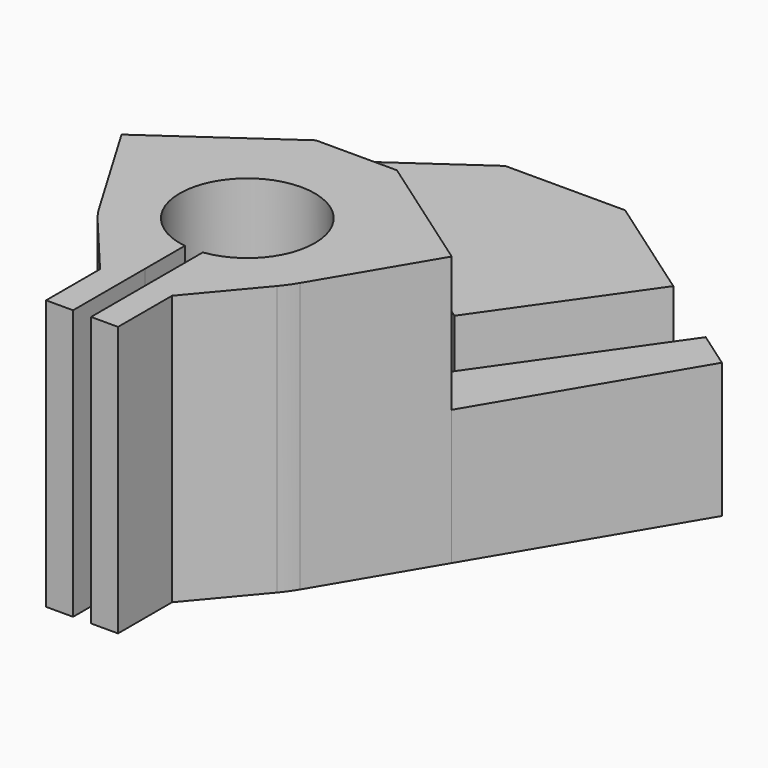
from build123d import *

# Parameters (mm, degrees)
F1_W     = 1.45
F1_H     = 6.3409252325
F2_DEPTH = 5
F3_DEPTH = 10
F5_DEPTH = 25
F6_DEPTH = 10
F4_R     = 0.725
F7_DEPTH = 32.664992266
F4_R_2   = 1.025
F8_DEPTH = 20.2234430885


# Not quite as in the source:
# - a feature names something its author has since deleted; it is built from what else it names


with BuildPart() as f2:
    # F1 (on Top) → F2 (new body)
    with BuildSketch(Plane.XY):
        with BuildLine():
            ThreePointArc((-21.8973851311, -18.9294214119), (-28.3829246015, -10.9960880786), (-20.899609828, -3.9960880786))
            ThreePointArc((-20.899609828, -3.9960880786), (-13.4162950544, -10.9960880786), (-19.9018345249, -18.9294214119))
            Line((-19.9018345249, -18.9294214119), (-19.9003497467, -24.4576265402))
            ThreePointArc((-19.9003497467, -24.4576265402), (-18.3828834375, -24.250149717), (-16.9003497467, -23.8656442066))
            ThreePointArc((-16.9003497467, -23.8656442066), (-13.6367119074, -22.2780319569), (-10.9391436703, -19.8500759839))
            ThreePointArc((-10.9391436703, -19.8500759839), (-10.2927451499, -19.0123651957), (-9.7166149372, -18.12486061))
            ThreePointArc((-9.7166149372, -18.12486061), (-9.4290474991, -5.3783924455), (-20.174609828, 1.4836798315))
            Line((-20.174609828, 1.4836798315), (-20.174609828, 0))
            Line((-20.174609828, 0), (-20.899609828, 0))
            Line((-20.899609828, 0), (-21.624609828, 0))
            Line((-21.624609828, 0), (-21.624609828, 1.4836798315))
            ThreePointArc((-21.624609828, 1.4836798315), (-32.3701721569, -5.3783924455), (-32.0826047188, -18.12486061))
            ThreePointArc((-32.0826047188, -18.12486061), (-31.5064745061, -19.0123651957), (-30.8600759857, -19.8500759839))
            ThreePointArc((-30.8600759857, -19.8500759839), (-28.1625077486, -22.2780319569), (-24.8988699093, -23.8656442066))
            ThreePointArc((-24.8988699093, -23.8656442066), (-23.4163362185, -24.250149717), (-21.8988699093, -24.4576265402))
            Line((-21.8988699093, -24.4576265402), (-21.8973851311, -18.9294214119))
        make_face()
        with BuildLine():
            Line((-21.8988699093, -34.4576265402), (-21.8988699093, -24.4576265402))
            ThreePointArc((-21.8988699093, -24.4576265402), (-23.4163362185, -24.250149717), (-24.8988699093, -23.8656442066))
            Line((-24.8988699093, -23.8656442066), (-24.8988699093, -26.9576265402))
            Line((-24.8988699093, -26.9576265402), (-24.8988699093, -34.4576265402))
            Line((-24.8988699093, -34.4576265402), (-21.8988699093, -34.4576265402))
        make_face()
        with BuildLine():
            ThreePointArc((-16.9003497467, -23.8656442066), (-18.3828834375, -24.250149717), (-19.9003497467, -24.4576265402))
            Line((-19.9003497467, -24.4576265402), (-19.9003497467, -34.4576265402))
            Line((-19.9003497467, -34.4576265402), (-16.9003497467, -34.4576265402))
            Line((-16.9003497467, -34.4576265402), (-16.9003497467, -26.9576265402))
            Line((-16.9003497467, -26.9576265402), (-16.9003497467, -23.8656442066))
        make_face()
        with BuildLine():
            Line((-24.8988699093, -26.9576265402), (-24.8988699093, -23.8656442066))
            ThreePointArc((-24.8988699093, -23.8656442066), (-28.1625077486, -22.2780319569), (-30.8600759857, -19.8500759839))
            Line((-30.8600759857, -19.8500759839), (-24.8988699093, -26.9576265402))
        make_face()
        with BuildLine():
            ThreePointArc((-10.9391436703, -19.8500759839), (-13.6367119074, -22.2780319569), (-16.9003497467, -23.8656442066))
            Line((-16.9003497467, -23.8656442066), (-16.9003497467, -26.9576265402))
            Line((-16.9003497467, -26.9576265402), (-10.9391436703, -19.8500759839))
        make_face()
        with BuildLine():
            Line((-39.2498481908, -6.0334444768), (-32.0826047188, -18.12486061))
            ThreePointArc((-32.0826047188, -18.12486061), (-32.3701721569, -5.3783924455), (-21.624609828, 1.4836798315))
            Line((-21.624609828, 1.4836798315), (-21.624609828, 3.6590747675))
            Line((-21.624609828, 3.6590747675), (-25.4074961518, 3.6590747675))
            Line((-25.4074961518, 3.6590747675), (-33.5990165947, -2.076689596))
            Line((-33.5990165947, -2.076689596), (-39.2498481908, -6.0334444768))
        make_face()
        with BuildLine():
            ThreePointArc((-20.174609828, 1.4836798315), (-9.4290474991, -5.3783924455), (-9.7166149372, -18.12486061))
            Line((-9.7166149372, -18.12486061), (-2.5493714652, -6.0334444768))
            Line((-2.5493714652, -6.0334444768), (-8.2002030613, -2.076689596))
            Line((-8.2002030613, -2.076689596), (-16.3917235042, 3.6590747675))
            Line((-16.3917235042, 3.6590747675), (-20.174609828, 3.6590747675))
            Line((-20.174609828, 3.6590747675), (-20.174609828, 1.4836798315))
        make_face()
        with BuildLine():
            Line((-21.624609828, 3.6590747675), (-21.624609828, 1.4836798315))
            ThreePointArc((-21.624609828, 1.4836798315), (-21.2622509514, 1.4988529145), (-20.899609828, 1.5039119214))
            ThreePointArc((-20.899609828, 1.5039119214), (-20.5369687046, 1.4988529145), (-20.174609828, 1.4836798315))
            Line((-20.174609828, 1.4836798315), (-20.174609828, 3.6590747675))
            Line((-20.174609828, 3.6590747675), (-21.624609828, 3.6590747675))
        make_face()
        with BuildLine():
            ThreePointArc((-20.899609828, 1.5039119214), (-21.2622509514, 1.4988529145), (-21.624609828, 1.4836798315))
            Line((-21.624609828, 1.4836798315), (-21.624609828, 0))
            Line((-21.624609828, 0), (-20.899609828, 0))
            Line((-20.899609828, 0), (-20.174609828, 0))
            Line((-20.174609828, 0), (-20.174609828, 1.4836798315))
            ThreePointArc((-20.174609828, 1.4836798315), (-20.5369687046, 1.4988529145), (-20.899609828, 1.5039119214))
        make_face()
        Polygon((-52.0341877249, 15.5342293294), (-39.2498481908, -6.0334444768), (-33.5990165947, -2.076689596), (-47.9384275035, 18.4021115112), align=None)
        Polygon((-8.2002030613, -2.076689596), (-2.5493714652, -6.0334444768), (10.2349680689, 15.5342293294), (6.1392078475, 18.4021115112), align=None)
        Polygon((-25.4074961518, 3.6590747675), (-21.624609828, 3.6590747675), (-21.624609828, 10), (-21.924609828, 10), (-27.2409219547, 6.2774781734), align=None)
        with Locations((-20.899609828, 6.8295373837)):
            Rectangle(F1_W, F1_H)
        Polygon((-47.9384275035, 18.4021115112), (-33.5990165947, -2.076689596), (-25.4074961518, 3.6590747675), (-27.2409219547, 6.2774781734), (-28.3880748274, 7.915782262), (-39.7469070606, 24.1378758747), align=None)
        Polygon((-16.3917235042, 3.6590747675), (-8.2002030613, -2.076689596), (6.1392078475, 18.4021115112), (-2.0523125954, 24.1378758747), (-13.4111448286, 7.915782262), (-14.5582977013, 6.2774781734), align=None)
        Polygon((-20.174609828, 10), (-20.174609828, 3.6590747675), (-16.3917235042, 3.6590747675), (-14.5582977013, 6.2774781734), (-19.874609828, 10), align=None)
        Polygon((-21.924609828, 10), (-21.624609828, 10), (-20.174609828, 10), (-19.874609828, 10), (-19.874609828, 12.4415491775), (-21.924609828, 12.4415491775), align=None)
        Polygon((-27.2409219547, 6.2774781734), (-21.924609828, 10), (-21.924609828, 12.4415491775), (-27.5689227831, 8.4893586983), (-28.3880748274, 7.915782262), align=None)
        Polygon((-38.9277550163, 24.7114523111), (-39.7469070606, 24.1378758747), (-28.3880748274, 7.915782262), (-27.5689227831, 8.4893586983), (-27.5689227831, 32.664992266), align=None)
        Polygon((-13.4111448286, 7.915782262), (-2.0523125954, 24.1378758747), (-2.8714646397, 24.7114523111), (-14.2302968729, 32.664992266), (-14.2302968729, 8.4893586983), align=None)
        Polygon((-19.874609828, 10), (-14.5582977013, 6.2774781734), (-13.4111448286, 7.915782262), (-14.2302968729, 8.4893586983), (-19.874609828, 12.4415491775), align=None)
        Polygon((-27.5689227831, 8.4893586983), (-21.924609828, 12.4415491775), (-21.924609828, 32.664992266), (-27.5689227831, 32.664992266), align=None)
        Polygon((-21.924609828, 32.664992266), (-21.924609828, 12.4415491775), (-19.874609828, 12.4415491775), (-19.874609828, 32.664992266), (-20.899609828, 32.664992266), align=None)
        Polygon((-19.874609828, 32.664992266), (-19.874609828, 12.4415491775), (-14.2302968729, 8.4893586983), (-14.2302968729, 32.664992266), align=None)
    extrude(amount=-F2_DEPTH)

    # F1 (on Top) → F5 (join)
    with BuildSketch(Plane.XY):
        with BuildLine():
            ThreePointArc((-21.8973851311, -18.9294214119), (-28.3829246015, -10.9960880786), (-20.899609828, -3.9960880786))
            ThreePointArc((-20.899609828, -3.9960880786), (-13.4162950544, -10.9960880786), (-19.9018345249, -18.9294214119))
            Line((-19.9018345249, -18.9294214119), (-19.9003497467, -24.4576265402))
            ThreePointArc((-19.9003497467, -24.4576265402), (-18.3828834375, -24.250149717), (-16.9003497467, -23.8656442066))
            ThreePointArc((-16.9003497467, -23.8656442066), (-13.6367119074, -22.2780319569), (-10.9391436703, -19.8500759839))
            ThreePointArc((-10.9391436703, -19.8500759839), (-10.2927451499, -19.0123651957), (-9.7166149372, -18.12486061))
            ThreePointArc((-9.7166149372, -18.12486061), (-9.4290474991, -5.3783924455), (-20.174609828, 1.4836798315))
            Line((-20.174609828, 1.4836798315), (-20.174609828, 0))
            Line((-20.174609828, 0), (-20.899609828, 0))
            Line((-20.899609828, 0), (-21.624609828, 0))
            Line((-21.624609828, 0), (-21.624609828, 1.4836798315))
            ThreePointArc((-21.624609828, 1.4836798315), (-32.3701721569, -5.3783924455), (-32.0826047188, -18.12486061))
            ThreePointArc((-32.0826047188, -18.12486061), (-31.5064745061, -19.0123651957), (-30.8600759857, -19.8500759839))
            ThreePointArc((-30.8600759857, -19.8500759839), (-28.1625077486, -22.2780319569), (-24.8988699093, -23.8656442066))
            ThreePointArc((-24.8988699093, -23.8656442066), (-23.4163362185, -24.250149717), (-21.8988699093, -24.4576265402))
            Line((-21.8988699093, -24.4576265402), (-21.8973851311, -18.9294214119))
        make_face()
        with BuildLine():
            Line((-21.8988699093, -34.4576265402), (-21.8988699093, -24.4576265402))
            ThreePointArc((-21.8988699093, -24.4576265402), (-23.4163362185, -24.250149717), (-24.8988699093, -23.8656442066))
            Line((-24.8988699093, -23.8656442066), (-24.8988699093, -26.9576265402))
            Line((-24.8988699093, -26.9576265402), (-24.8988699093, -34.4576265402))
            Line((-24.8988699093, -34.4576265402), (-21.8988699093, -34.4576265402))
        make_face()
        with BuildLine():
            ThreePointArc((-16.9003497467, -23.8656442066), (-18.3828834375, -24.250149717), (-19.9003497467, -24.4576265402))
            Line((-19.9003497467, -24.4576265402), (-19.9003497467, -34.4576265402))
            Line((-19.9003497467, -34.4576265402), (-16.9003497467, -34.4576265402))
            Line((-16.9003497467, -34.4576265402), (-16.9003497467, -26.9576265402))
            Line((-16.9003497467, -26.9576265402), (-16.9003497467, -23.8656442066))
        make_face()
        with BuildLine():
            Line((-24.8988699093, -26.9576265402), (-24.8988699093, -23.8656442066))
            ThreePointArc((-24.8988699093, -23.8656442066), (-28.1625077486, -22.2780319569), (-30.8600759857, -19.8500759839))
            Line((-30.8600759857, -19.8500759839), (-24.8988699093, -26.9576265402))
        make_face()
        with BuildLine():
            ThreePointArc((-10.9391436703, -19.8500759839), (-13.6367119074, -22.2780319569), (-16.9003497467, -23.8656442066))
            Line((-16.9003497467, -23.8656442066), (-16.9003497467, -26.9576265402))
            Line((-16.9003497467, -26.9576265402), (-10.9391436703, -19.8500759839))
        make_face()
        with BuildLine():
            Line((-39.2498481908, -6.0334444768), (-32.0826047188, -18.12486061))
            ThreePointArc((-32.0826047188, -18.12486061), (-32.3701721569, -5.3783924455), (-21.624609828, 1.4836798315))
            Line((-21.624609828, 1.4836798315), (-21.624609828, 3.6590747675))
            Line((-21.624609828, 3.6590747675), (-25.4074961518, 3.6590747675))
            Line((-25.4074961518, 3.6590747675), (-33.5990165947, -2.076689596))
            Line((-33.5990165947, -2.076689596), (-39.2498481908, -6.0334444768))
        make_face()
        with BuildLine():
            ThreePointArc((-20.174609828, 1.4836798315), (-9.4290474991, -5.3783924455), (-9.7166149372, -18.12486061))
            Line((-9.7166149372, -18.12486061), (-2.5493714652, -6.0334444768))
            Line((-2.5493714652, -6.0334444768), (-8.2002030613, -2.076689596))
            Line((-8.2002030613, -2.076689596), (-16.3917235042, 3.6590747675))
            Line((-16.3917235042, 3.6590747675), (-20.174609828, 3.6590747675))
            Line((-20.174609828, 3.6590747675), (-20.174609828, 1.4836798315))
        make_face()
        with BuildLine():
            Line((-21.624609828, 3.6590747675), (-21.624609828, 1.4836798315))
            ThreePointArc((-21.624609828, 1.4836798315), (-21.2622509514, 1.4988529145), (-20.899609828, 1.5039119214))
            ThreePointArc((-20.899609828, 1.5039119214), (-20.5369687046, 1.4988529145), (-20.174609828, 1.4836798315))
            Line((-20.174609828, 1.4836798315), (-20.174609828, 3.6590747675))
            Line((-20.174609828, 3.6590747675), (-21.624609828, 3.6590747675))
        make_face()
        with BuildLine():
            ThreePointArc((-20.899609828, 1.5039119214), (-21.2622509514, 1.4988529145), (-21.624609828, 1.4836798315))
            Line((-21.624609828, 1.4836798315), (-21.624609828, 0))
            Line((-21.624609828, 0), (-20.899609828, 0))
            Line((-20.899609828, 0), (-20.174609828, 0))
            Line((-20.174609828, 0), (-20.174609828, 1.4836798315))
            ThreePointArc((-20.174609828, 1.4836798315), (-20.5369687046, 1.4988529145), (-20.899609828, 1.5039119214))
        make_face()
    extrude(amount=F5_DEPTH)

    # F1 (on Top) → F6 (join)
    with BuildSketch(Plane.XY):
        with BuildLine():
            ThreePointArc((-21.8973851311, -18.9294214119), (-28.3829246015, -10.9960880786), (-20.899609828, -3.9960880786))
            ThreePointArc((-20.899609828, -3.9960880786), (-13.4162950544, -10.9960880786), (-19.9018345249, -18.9294214119))
            Line((-19.9018345249, -18.9294214119), (-19.9003497467, -24.4576265402))
            ThreePointArc((-19.9003497467, -24.4576265402), (-18.3828834375, -24.250149717), (-16.9003497467, -23.8656442066))
            ThreePointArc((-16.9003497467, -23.8656442066), (-13.6367119074, -22.2780319569), (-10.9391436703, -19.8500759839))
            ThreePointArc((-10.9391436703, -19.8500759839), (-10.2927451499, -19.0123651957), (-9.7166149372, -18.12486061))
            ThreePointArc((-9.7166149372, -18.12486061), (-9.4290474991, -5.3783924455), (-20.174609828, 1.4836798315))
            Line((-20.174609828, 1.4836798315), (-20.174609828, 0))
            Line((-20.174609828, 0), (-20.899609828, 0))
            Line((-20.899609828, 0), (-21.624609828, 0))
            Line((-21.624609828, 0), (-21.624609828, 1.4836798315))
            ThreePointArc((-21.624609828, 1.4836798315), (-32.3701721569, -5.3783924455), (-32.0826047188, -18.12486061))
            ThreePointArc((-32.0826047188, -18.12486061), (-31.5064745061, -19.0123651957), (-30.8600759857, -19.8500759839))
            ThreePointArc((-30.8600759857, -19.8500759839), (-28.1625077486, -22.2780319569), (-24.8988699093, -23.8656442066))
            ThreePointArc((-24.8988699093, -23.8656442066), (-23.4163362185, -24.250149717), (-21.8988699093, -24.4576265402))
            Line((-21.8988699093, -24.4576265402), (-21.8973851311, -18.9294214119))
        make_face()
        with BuildLine():
            Line((-24.8988699093, -26.9576265402), (-24.8988699093, -23.8656442066))
            ThreePointArc((-24.8988699093, -23.8656442066), (-28.1625077486, -22.2780319569), (-30.8600759857, -19.8500759839))
            Line((-30.8600759857, -19.8500759839), (-24.8988699093, -26.9576265402))
        make_face()
        with BuildLine():
            Line((-21.8988699093, -34.4576265402), (-21.8988699093, -24.4576265402))
            ThreePointArc((-21.8988699093, -24.4576265402), (-23.4163362185, -24.250149717), (-24.8988699093, -23.8656442066))
            Line((-24.8988699093, -23.8656442066), (-24.8988699093, -26.9576265402))
            Line((-24.8988699093, -26.9576265402), (-24.8988699093, -34.4576265402))
            Line((-24.8988699093, -34.4576265402), (-21.8988699093, -34.4576265402))
        make_face()
        with BuildLine():
            ThreePointArc((-16.9003497467, -23.8656442066), (-18.3828834375, -24.250149717), (-19.9003497467, -24.4576265402))
            Line((-19.9003497467, -24.4576265402), (-19.9003497467, -34.4576265402))
            Line((-19.9003497467, -34.4576265402), (-16.9003497467, -34.4576265402))
            Line((-16.9003497467, -34.4576265402), (-16.9003497467, -26.9576265402))
            Line((-16.9003497467, -26.9576265402), (-16.9003497467, -23.8656442066))
        make_face()
        with BuildLine():
            ThreePointArc((-10.9391436703, -19.8500759839), (-13.6367119074, -22.2780319569), (-16.9003497467, -23.8656442066))
            Line((-16.9003497467, -23.8656442066), (-16.9003497467, -26.9576265402))
            Line((-16.9003497467, -26.9576265402), (-10.9391436703, -19.8500759839))
        make_face()
        Polygon((-52.0341877249, 15.5342293294), (-39.2498481908, -6.0334444768), (-33.5990165947, -2.076689596), (-47.9384275035, 18.4021115112), align=None)
        Polygon((-8.2002030613, -2.076689596), (-2.5493714652, -6.0334444768), (10.2349680689, 15.5342293294), (6.1392078475, 18.4021115112), align=None)
        with BuildLine():
            Line((-39.2498481908, -6.0334444768), (-32.0826047188, -18.12486061))
            ThreePointArc((-32.0826047188, -18.12486061), (-32.3701721569, -5.3783924455), (-21.624609828, 1.4836798315))
            Line((-21.624609828, 1.4836798315), (-21.624609828, 3.6590747675))
            Line((-21.624609828, 3.6590747675), (-25.4074961518, 3.6590747675))
            Line((-25.4074961518, 3.6590747675), (-33.5990165947, -2.076689596))
            Line((-33.5990165947, -2.076689596), (-39.2498481908, -6.0334444768))
        make_face()
        with BuildLine():
            ThreePointArc((-20.174609828, 1.4836798315), (-9.4290474991, -5.3783924455), (-9.7166149372, -18.12486061))
            Line((-9.7166149372, -18.12486061), (-2.5493714652, -6.0334444768))
            Line((-2.5493714652, -6.0334444768), (-8.2002030613, -2.076689596))
            Line((-8.2002030613, -2.076689596), (-16.3917235042, 3.6590747675))
            Line((-16.3917235042, 3.6590747675), (-20.174609828, 3.6590747675))
            Line((-20.174609828, 3.6590747675), (-20.174609828, 1.4836798315))
        make_face()
        with BuildLine():
            ThreePointArc((-20.899609828, 1.5039119214), (-21.2622509514, 1.4988529145), (-21.624609828, 1.4836798315))
            Line((-21.624609828, 1.4836798315), (-21.624609828, 0))
            Line((-21.624609828, 0), (-20.899609828, 0))
            Line((-20.899609828, 0), (-20.174609828, 0))
            Line((-20.174609828, 0), (-20.174609828, 1.4836798315))
            ThreePointArc((-20.174609828, 1.4836798315), (-20.5369687046, 1.4988529145), (-20.899609828, 1.5039119214))
        make_face()
        Polygon((-20.174609828, 10), (-20.174609828, 3.6590747675), (-16.3917235042, 3.6590747675), (-14.5582977013, 6.2774781734), (-19.874609828, 10), align=None)
        Polygon((-25.4074961518, 3.6590747675), (-21.624609828, 3.6590747675), (-21.624609828, 10), (-21.924609828, 10), (-27.2409219547, 6.2774781734), align=None)
        with Locations((-20.899609828, 6.8295373837)):
            Rectangle(F1_W, F1_H)
    extrude(amount=F6_DEPTH)


with BuildPart() as f3:
    # F1 (on Top) → F3 (new body)
    with BuildSketch(Plane.XY):
        Polygon((-19.874609828, 32.664992266), (-19.874609828, 12.4415491775), (-14.2302968729, 8.4893586983), (-14.2302968729, 32.664992266), align=None)
        Polygon((-27.5689227831, 8.4893586983), (-21.924609828, 12.4415491775), (-21.924609828, 32.664992266), (-27.5689227831, 32.664992266), align=None)
        Polygon((-38.9277550163, 24.7114523111), (-39.7469070606, 24.1378758747), (-28.3880748274, 7.915782262), (-27.5689227831, 8.4893586983), (-27.5689227831, 32.664992266), align=None)
        Polygon((-13.4111448286, 7.915782262), (-2.0523125954, 24.1378758747), (-2.8714646397, 24.7114523111), (-14.2302968729, 32.664992266), (-14.2302968729, 8.4893586983), align=None)
        Polygon((-21.924609828, 32.664992266), (-21.924609828, 12.4415491775), (-19.874609828, 12.4415491775), (-19.874609828, 32.664992266), (-20.899609828, 32.664992266), align=None)
    extrude(amount=F3_DEPTH)


with BuildPart() as f7_tool:
    # F4 (on face) → F7 (new body, through all)
    with BuildSketch(Plane(origin=(0, 32.664992266, 0), x_dir=(-1, 0, 0), z_dir=(0, 1, 0))):
        with Locations((20.899609828, 5)):
            Circle(F4_R)
    extrude(amount=-F7_DEPTH)


with BuildPart() as f2_1:
    add(f2.part)

    # F7: cut by f7_tool
    add(f7_tool.part, mode=Mode.SUBTRACT)


with BuildPart() as f3_1:
    add(f3.part)

    # F7: cut by f7_tool
    add(f7_tool.part, mode=Mode.SUBTRACT)

    # F4 (on face) → F8 (cut, through all)
    with BuildSketch(Plane(origin=(0, 32.664992266, 0), x_dir=(-1, 0, 0), z_dir=(0, 1, 0))):
        with Locations((20.899609828, 5)):
            Circle(F4_R_2)
        with Locations((20.899609828, 5)):
            Circle(F4_R, mode=Mode.SUBTRACT)
    extrude(amount=-F8_DEPTH, mode=Mode.SUBTRACT)


solid = Compound([f2_1.part, f3_1.part])
